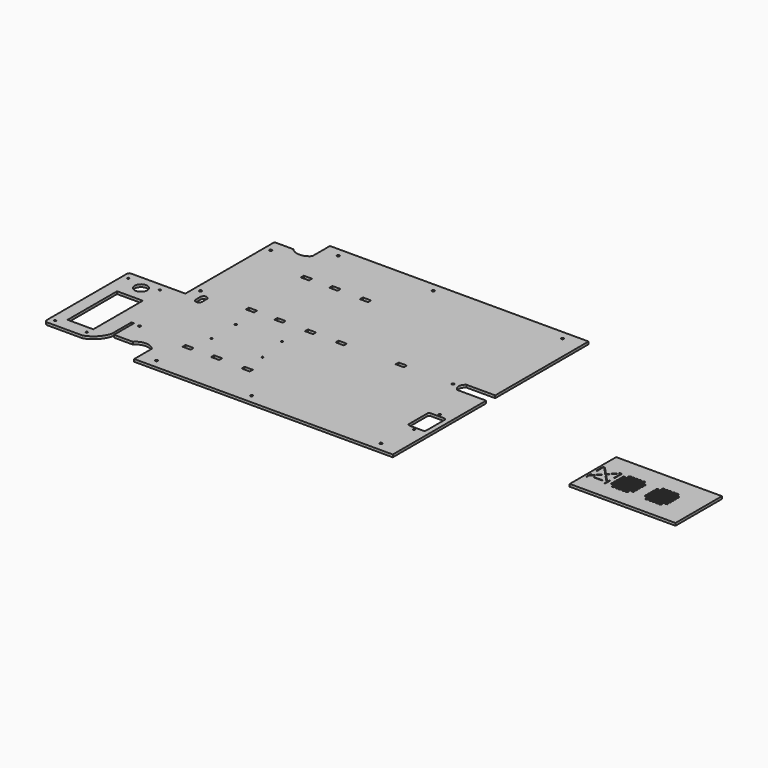
from build123d import *

# Parameters (mm, degrees)
F0_R     = 1.5
F0_R_2   = 2
F0_W     = 40.723241355
F0_H     = 98.1378996708
F0_W_2   = 13
F0_H_2   = 6
F0_R_3   = 10
F1_DEPTH = 4
F0_W_3   = 167.7038488136
F0_H_3   = 92
F0_W_4   = 13.1770956796
F0_H_4   = 1


# Not quite as in the source:
# - a feature names something its author has since deleted; it is built from what else it names


with BuildPart() as f1:
    # F0 (on Top) → F1 (new body)
    with BuildSketch(Plane.XY):
        with BuildLine():
            Line((235, 20), (235, 190))
            Line((235, 190), (235, 194))
            Line((235, 194), (160.2169722319, 194))
            Line((160.2169722319, 194), (-175, 194))
            Line((-175, 194), (-175, 159))
            ThreePointArc((-175, 159), (-190, 152.2242824696), (-205, 159))
            Line((-205, 159), (-235, 159))
            Line((-235, 159), (-235, 18))
            Line((-235, 18), (-235, 0))
            Line((-235, 0), (-235, -17.580891105))
            Line((-235, -17.580891105), (-322.3694663308, -17.580891105))
            ThreePointArc((-322.3694663308, -17.580891105), (-324.1034075985, -19.3986567512), (-324.7344900249, -21.8302322148))
            Line((-324.7344900249, -21.8302322148), (-324.7344900249, -179.7310591129))
            ThreePointArc((-324.7344900249, -179.7310591129), (-323.2700239308, -183.2665930188), (-319.7344900249, -184.7310591129))
            Line((-319.7344900249, -184.7310591129), (-264.2700470778, -184.7310591129))
            ThreePointArc((-264.2700470778, -184.7310591129), (-248.5516048539, -174.8937039891), (-239, -159))
            Line((-239, -159), (-239, -119.5373386145))
            Line((-239, -119.5373386145), (-235, -119.5373386145))
            Line((-235, -119.5373386145), (-235, -141))
            Line((-235, -141), (-235, -141.1135244755))
            Line((-235, -141.1135244755), (-235, -159))
            Line((-235, -159), (-205, -159))
            ThreePointArc((-205, -159), (-190, -152.2242824696), (-175, -159))
            Line((-175, -159), (-175, -194))
            Line((-175, -194), (160.2169722319, -194))
            Line((160.2169722319, -194), (235, -194))
            Line((235, -194), (235, -190))
            Line((235, -190), (235, -20))
            Line((235, -20), (235, -9))
            Line((235, -9), (189.4401907921, -9))
            ThreePointArc((189.4401907921, -9), (184.4617959967, 0), (189.4401907921, 9))
            Line((189.4401907921, 9), (235, 9))
            Line((235, 9), (235, 20))
        make_face()
        with Locations((-315.7939992134, -174.6363174207)):
            Circle(F0_R, mode=Mode.SUBTRACT)
        with Locations((-265.8466312134, -174.8205274207)):
            Circle(F0_R, mode=Mode.SUBTRACT)
        with Locations((-150.6642103195, -180)):
            Circle(F0_R_2, mode=Mode.SUBTRACT)
        with Locations((-284.6316677553, -114.4722954954)):
            Rectangle(F0_W, F0_H, mode=Mode.SUBTRACT)
        with Locations((-225, -121)):
            Circle(F0_R_2, mode=Mode.SUBTRACT)
        with Locations((-142.3513439298, -128.0134530067)):
            Rectangle(F0_W_2, F0_H_2, mode=Mode.SUBTRACT)
        with Locations((-97.480445087, -127.4769221544)):
            Rectangle(F0_W_2, F0_H_2, mode=Mode.SUBTRACT)
        with Locations((0, -180)):
            Circle(F0_R_2, mode=Mode.SUBTRACT)
        with Locations((-48.8024120331, -127.8542791605)):
            Rectangle(F0_W_2, F0_H_2, mode=Mode.SUBTRACT)
        with Locations((-134.561391694, -91.3646608818)):
            Circle(F0_R, mode=Mode.SUBTRACT)
        with Locations((-287.3536279337, -40.1161199984)):
            Circle(F0_R_3, mode=Mode.SUBTRACT)
        with Locations((-315.8466312134, -29.6363174207)):
            Circle(F0_R, mode=Mode.SUBTRACT)
        with Locations((-265.8466312134, -29.6363174207)):
            Circle(F0_R, mode=Mode.SUBTRACT)
        with BuildLine():
            ThreePointArc((-215, -12.7703770995), (-210, -7.7703770995), (-205, -12.7703770995))
            Line((-205, -12.7703770995), (-205, -21.7703770995))
            ThreePointArc((-205, -21.7703770995), (-210, -26.7703770995), (-215, -21.7703770995))
            Line((-215, -21.7703770995), (-215, -12.7703770995))
        make_face(mode=Mode.SUBTRACT)
        with BuildLine():
            ThreePointArc((-223, 0), (-225, -2), (-227, 0))
            ThreePointArc((-227, 0), (-225, 2), (-223, 0))
        make_face(mode=Mode.SUBTRACT)
        with Locations((-134.564578694, -43.3323348818)):
            Circle(F0_R, mode=Mode.SUBTRACT)
        with Locations((-143.6203961174, -0.9194955441)):
            Rectangle(F0_W_2, F0_H_2, mode=Mode.SUBTRACT)
        with Locations((-98.7494972746, -0.3829646918)):
            Rectangle(F0_W_2, F0_H_2, mode=Mode.SUBTRACT)
        with Locations((-53.852118694, -91.0625058818)):
            Circle(F0_R, mode=Mode.SUBTRACT)
        with Locations((-61.225924694, -43.2365928818)):
            Circle(F0_R, mode=Mode.SUBTRACT)
        with Locations((-50.0714642207, -0.7603216978)):
            Rectangle(F0_W_2, F0_H_2, mode=Mode.SUBTRACT)
        with Locations((-1.5765217012, -0.5216977205)):
            Rectangle(F0_W_2, F0_H_2, mode=Mode.SUBTRACT)
        with Locations((205, -180)):
            Circle(F0_R_2, mode=Mode.SUBTRACT)
        with Locations((213.4276428699, -125)):
            Circle(F0_R, mode=Mode.SUBTRACT)
        with BuildLine():
            Line((199.6276428699, -117.6), (199.6276428699, -81.4))
            ThreePointArc((199.6276428699, -81.4), (200.5063225264, -79.2786796564), (202.6276428699, -78.4))
            Line((202.6276428699, -78.4), (224.2276428699, -78.4))
            ThreePointArc((224.2276428699, -78.4), (226.3489632135, -79.2786796564), (227.2276428699, -81.4))
            Line((227.2276428699, -81.4), (227.2276428699, -117.6))
            ThreePointArc((227.2276428699, -117.6), (226.3489632135, -119.7213203436), (224.2276428699, -120.6))
            Line((224.2276428699, -120.6), (202.6276428699, -120.6))
            ThreePointArc((202.6276428699, -120.6), (200.5063225264, -119.7213203436), (199.6276428699, -117.6))
        make_face(mode=Mode.SUBTRACT)
        with Locations((213.4276428699, -74)):
            Circle(F0_R, mode=Mode.SUBTRACT)
        with Locations((175, 0)):
            Circle(F0_R_2, mode=Mode.SUBTRACT)
        with Locations((93.1805941164, 0.1503385957)):
            Rectangle(F0_W_2, F0_H_2, mode=Mode.SUBTRACT)
        with Locations((-225, 139)):
            Circle(F0_R_2, mode=Mode.SUBTRACT)
        with Locations((-143.9774875442, 108.5958170493)):
            Rectangle(F0_W_2, F0_H_2, mode=Mode.SUBTRACT)
        with Locations((-99.1065887014, 109.1323479017)):
            Rectangle(F0_W_2, F0_H_2, mode=Mode.SUBTRACT)
        with Locations((-150.6642103195, 180)):
            Circle(F0_R_2, mode=Mode.SUBTRACT)
        with Locations((-50.4285556475, 108.7549908956)):
            Rectangle(F0_W_2, F0_H_2, mode=Mode.SUBTRACT)
        with Locations((0, 180)):
            Circle(F0_R_2, mode=Mode.SUBTRACT)
        with Locations((205, 180)):
            Circle(F0_R_2, mode=Mode.SUBTRACT)
    extrude(amount=F1_DEPTH)


with BuildPart() as f1b:
    # F0 (on Top) → F1, piece 2 (new body)
    with BuildSketch(Plane.XY):
        with Locations((539.1946978695, -72.6823304409)):
            Rectangle(F0_W_3, F0_H_3)
        with Locations((474.1243227663, -86.1302117599)):
            Rectangle(F0_W_4, F0_H_4, mode=Mode.SUBTRACT)
        Polygon((499.6697502675, -90.1), (500.8244508059, -88.1), (503.1338518827, -88.1), (504.2885524211, -90.1), (503.1338518827, -92.1), (500.8244508059, -92.1), align=None, mode=Mode.SUBTRACT)
        Polygon((470.3372043136, -74.1853925354), (471.1485323172, -74.7817042836), (460.0899253393, -86.6302117599), (460.0899253393, -90.7567794457), (459.0899253393, -90.7567794457), (459.0899253393, -86.2360485793), (459.0899253393, -80.9347892446), (460.0899253393, -80.9347892446), (460.0899253393, -85.1646200079), align=None, mode=Mode.SUBTRACT)
        Polygon((488.0899253393, -86.6302117599), (477.0313183614, -74.7817042836), (477.8426463649, -74.1853925354), (488.0899253393, -85.1646200079), (488.0899253393, -80.9347892446), (489.0899253393, -80.9347892446), (489.0899253393, -86.2360485793), (489.0899253393, -90.7567794457), (488.0899253393, -90.7567794457), align=None, mode=Mode.SUBTRACT)
        Polygon((494.3197502675, -84.75), (495.4744508059, -82.75), (497.7838518827, -82.75), (498.9385524211, -84.75), (497.7838518827, -86.75), (495.4744508059, -86.75), align=None, mode=Mode.SUBTRACT)
        Polygon((499.6697502675, -84.75), (500.8244508059, -82.75), (503.1338518827, -82.75), (504.2885524211, -84.75), (503.1338518827, -86.75), (500.8244508059, -86.75), align=None, mode=Mode.SUBTRACT)
        Polygon((494.3197502675, -79.4), (495.4744508059, -77.4), (497.7838518827, -77.4), (498.9385524211, -79.4), (497.7838518827, -81.4), (495.4744508059, -81.4), align=None, mode=Mode.SUBTRACT)
        Polygon((499.6697502675, -79.4), (500.8244508059, -77.4), (503.1338518827, -77.4), (504.2885524211, -79.4), (503.1338518827, -81.4), (500.8244508059, -81.4), align=None, mode=Mode.SUBTRACT)
        Polygon((494.3197502675, -74.05), (495.4744508059, -72.05), (497.7838518827, -72.05), (498.9385524211, -74.05), (497.7838518827, -76.05), (495.4744508059, -76.05), align=None, mode=Mode.SUBTRACT)
        Polygon((499.6697502675, -74.05), (500.8244508059, -72.05), (503.1338518827, -72.05), (504.2885524211, -74.05), (503.1338518827, -76.05), (500.8244508059, -76.05), align=None, mode=Mode.SUBTRACT)
        with BuildLine():
            Line((474.0899253393, -71.6302117599), (461.8209806075, -58.484913833))
            ThreePointArc((461.8209806075, -58.484913833), (460.7232205999, -58.2368947069), (460.0899253393, -59.1672320834))
            Line((460.0899253393, -59.1672320834), (460.0899253393, -71.6302117599))
            Line((460.0899253393, -71.6302117599), (459.0899253393, -71.6302117599))
            Line((459.0899253393, -71.6302117599), (459.0899253393, -59.1672320834))
            ThreePointArc((459.0899253393, -59.1672320834), (460.3565158605, -57.3065573304), (462.5520358758, -57.8025955827))
            Line((462.5520358758, -57.8025955827), (474.0899253393, -70.1646200079))
            Line((474.0899253393, -70.1646200079), (485.6278148028, -57.8025955827))
            ThreePointArc((485.6278148028, -57.8025955827), (487.823334818, -57.3065573304), (489.0899253393, -59.1672320834))
            Line((489.0899253393, -59.1672320834), (489.0899253393, -71.6302117599))
            Line((489.0899253393, -71.6302117599), (488.0899253393, -71.6302117599))
            Line((488.0899253393, -71.6302117599), (488.0899253393, -59.1672320834))
            ThreePointArc((488.0899253393, -59.1672320834), (487.4566300786, -58.2368947069), (486.358870071, -58.484913833))
            Line((486.358870071, -58.484913833), (474.0899253393, -71.6302117599))
        make_face(mode=Mode.SUBTRACT)
        Polygon((494.3197502675, -68.7), (495.4744508059, -66.7), (497.7838518827, -66.7), (498.9385524211, -68.7), (497.7838518827, -70.7), (495.4744508059, -70.7), align=None, mode=Mode.SUBTRACT)
        Polygon((499.6697502675, -68.7), (500.8244508059, -66.7), (503.1338518827, -66.7), (504.2885524211, -68.7), (503.1338518827, -70.7), (500.8244508059, -70.7), align=None, mode=Mode.SUBTRACT)
        Polygon((494.3197502675, -63.35), (495.4744508059, -61.35), (497.7838518827, -61.35), (498.9385524211, -63.35), (497.7838518827, -65.35), (495.4744508059, -65.35), align=None, mode=Mode.SUBTRACT)
        Polygon((499.6697502675, -63.35), (500.8244508059, -61.35), (503.1338518827, -61.35), (504.2885524211, -63.35), (503.1338518827, -65.35), (500.8244508059, -65.35), align=None, mode=Mode.SUBTRACT)
        Polygon((499.6697502675, -58), (500.8244508059, -56), (503.1338518827, -56), (504.2885524211, -58), (503.1338518827, -60), (500.8244508059, -60), align=None, mode=Mode.SUBTRACT)
        Polygon((505.0197502675, -90.1), (506.1744508059, -88.1), (508.4838518827, -88.1), (509.6385524211, -90.1), (508.4838518827, -92.1), (506.1744508059, -92.1), align=None, mode=Mode.SUBTRACT)
        Polygon((510.3697502675, -90.1), (511.5244508059, -88.1), (513.8338518827, -88.1), (514.9885524211, -90.1), (513.8338518827, -92.1), (511.5244508059, -92.1), align=None, mode=Mode.SUBTRACT)
        Polygon((515.7197502675, -90.1), (516.8744508059, -88.1), (519.1838518827, -88.1), (520.3385524211, -90.1), (519.1838518827, -92.1), (516.8744508059, -92.1), align=None, mode=Mode.SUBTRACT)
        Polygon((521.0697502675, -90.1), (522.2244508059, -88.1), (524.5338518827, -88.1), (525.6885524211, -90.1), (524.5338518827, -92.1), (522.2244508059, -92.1), align=None, mode=Mode.SUBTRACT)
        Polygon((557.1102443947, -91.2547005384), (555.1102443947, -92.4094010768), (553.1102443947, -91.2547005384), (553.1102443947, -88.9452994616), (555.1102443947, -87.7905989232), (557.1102443947, -88.9452994616), align=None, mode=Mode.SUBTRACT)
        Polygon((562.4602443947, -91.2547005384), (560.4602443947, -92.4094010768), (558.4602443947, -91.2547005384), (558.4602443947, -88.9452994616), (560.4602443947, -87.7905989232), (562.4602443947, -88.9452994616), align=None, mode=Mode.SUBTRACT)
        Polygon((505.0197502675, -84.75), (506.1744508059, -82.75), (508.4838518827, -82.75), (509.6385524211, -84.75), (508.4838518827, -86.75), (506.1744508059, -86.75), align=None, mode=Mode.SUBTRACT)
        Polygon((510.3697502675, -84.75), (511.5244508059, -82.75), (513.8338518827, -82.75), (514.9885524211, -84.75), (513.8338518827, -86.75), (511.5244508059, -86.75), align=None, mode=Mode.SUBTRACT)
        Polygon((515.7197502675, -84.75), (516.8744508059, -82.75), (519.1838518827, -82.75), (520.3385524211, -84.75), (519.1838518827, -86.75), (516.8744508059, -86.75), align=None, mode=Mode.SUBTRACT)
        Polygon((505.0197502675, -79.4), (506.1744508059, -77.4), (508.4838518827, -77.4), (509.6385524211, -79.4), (508.4838518827, -81.4), (506.1744508059, -81.4), align=None, mode=Mode.SUBTRACT)
        Polygon((510.3697502675, -79.4), (511.5244508059, -77.4), (513.8338518827, -77.4), (514.9885524211, -79.4), (513.8338518827, -81.4), (511.5244508059, -81.4), align=None, mode=Mode.SUBTRACT)
        Polygon((515.7197502675, -79.4), (516.8744508059, -77.4), (519.1838518827, -77.4), (520.3385524211, -79.4), (519.1838518827, -81.4), (516.8744508059, -81.4), align=None, mode=Mode.SUBTRACT)
        Polygon((521.0697502675, -84.75), (522.2244508059, -82.75), (524.5338518827, -82.75), (525.6885524211, -84.75), (524.5338518827, -86.75), (522.2244508059, -86.75), align=None, mode=Mode.SUBTRACT)
        Polygon((526.4197502675, -84.75), (527.5744508059, -82.75), (529.8838518827, -82.75), (531.0385524211, -84.75), (529.8838518827, -86.75), (527.5744508059, -86.75), align=None, mode=Mode.SUBTRACT)
        Polygon((521.0697502675, -79.4), (522.2244508059, -77.4), (524.5338518827, -77.4), (525.6885524211, -79.4), (524.5338518827, -81.4), (522.2244508059, -81.4), align=None, mode=Mode.SUBTRACT)
        Polygon((526.4197502675, -79.4), (527.5744508059, -77.4), (529.8838518827, -77.4), (531.0385524211, -79.4), (529.8838518827, -81.4), (527.5744508059, -81.4), align=None, mode=Mode.SUBTRACT)
        Polygon((505.0197502675, -74.05), (506.1744508059, -72.05), (508.4838518827, -72.05), (509.6385524211, -74.05), (508.4838518827, -76.05), (506.1744508059, -76.05), align=None, mode=Mode.SUBTRACT)
        Polygon((510.3697502675, -74.05), (511.5244508059, -72.05), (513.8338518827, -72.05), (514.9885524211, -74.05), (513.8338518827, -76.05), (511.5244508059, -76.05), align=None, mode=Mode.SUBTRACT)
        Polygon((515.7197502675, -74.05), (516.8744508059, -72.05), (519.1838518827, -72.05), (520.3385524211, -74.05), (519.1838518827, -76.05), (516.8744508059, -76.05), align=None, mode=Mode.SUBTRACT)
        Polygon((521.0697502675, -74.05), (522.2244508059, -72.05), (524.5338518827, -72.05), (525.6885524211, -74.05), (524.5338518827, -76.05), (522.2244508059, -76.05), align=None, mode=Mode.SUBTRACT)
        Polygon((526.4197502675, -74.05), (527.5744508059, -72.05), (529.8838518827, -72.05), (531.0385524211, -74.05), (529.8838518827, -76.05), (527.5744508059, -76.05), align=None, mode=Mode.SUBTRACT)
        Polygon((551.7602443947, -85.9047005384), (549.7602443947, -87.0594010768), (547.7602443947, -85.9047005384), (547.7602443947, -83.5952994616), (549.7602443947, -82.4405989232), (551.7602443947, -83.5952994616), align=None, mode=Mode.SUBTRACT)
        Polygon((557.1102443947, -85.9047005384), (555.1102443947, -87.0594010768), (553.1102443947, -85.9047005384), (553.1102443947, -83.5952994616), (555.1102443947, -82.4405989232), (557.1102443947, -83.5952994616), align=None, mode=Mode.SUBTRACT)
        Polygon((562.4602443947, -85.9047005384), (560.4602443947, -87.0594010768), (558.4602443947, -85.9047005384), (558.4602443947, -83.5952994616), (560.4602443947, -82.4405989232), (562.4602443947, -83.5952994616), align=None, mode=Mode.SUBTRACT)
        Polygon((551.7602443947, -80.5547005384), (549.7602443947, -81.7094010768), (547.7602443947, -80.5547005384), (547.7602443947, -78.2452994616), (549.7602443947, -77.0905989232), (551.7602443947, -78.2452994616), align=None, mode=Mode.SUBTRACT)
        Polygon((557.1102443947, -80.5547005384), (555.1102443947, -81.7094010768), (553.1102443947, -80.5547005384), (553.1102443947, -78.2452994616), (555.1102443947, -77.0905989232), (557.1102443947, -78.2452994616), align=None, mode=Mode.SUBTRACT)
        Polygon((562.4602443947, -80.5547005384), (560.4602443947, -81.7094010768), (558.4602443947, -80.5547005384), (558.4602443947, -78.2452994616), (560.4602443947, -77.0905989232), (562.4602443947, -78.2452994616), align=None, mode=Mode.SUBTRACT)
        Polygon((551.7602443947, -75.2047005384), (549.7602443947, -76.3594010768), (547.7602443947, -75.2047005384), (547.7602443947, -72.8952994616), (549.7602443947, -71.7405989232), (551.7602443947, -72.8952994616), align=None, mode=Mode.SUBTRACT)
        Polygon((557.1102443947, -75.2047005384), (555.1102443947, -76.3594010768), (553.1102443947, -75.2047005384), (553.1102443947, -72.8952994616), (555.1102443947, -71.7405989232), (557.1102443947, -72.8952994616), align=None, mode=Mode.SUBTRACT)
        Polygon((562.4602443947, -75.2047005384), (560.4602443947, -76.3594010768), (558.4602443947, -75.2047005384), (558.4602443947, -72.8952994616), (560.4602443947, -71.7405989232), (562.4602443947, -72.8952994616), align=None, mode=Mode.SUBTRACT)
        Polygon((567.8102443947, -91.2547005384), (565.8102443947, -92.4094010768), (563.8102443947, -91.2547005384), (563.8102443947, -88.9452994616), (565.8102443947, -87.7905989232), (567.8102443947, -88.9452994616), align=None, mode=Mode.SUBTRACT)
        Polygon((573.1602443947, -91.2547005384), (571.1602443947, -92.4094010768), (569.1602443947, -91.2547005384), (569.1602443947, -88.9452994616), (571.1602443947, -87.7905989232), (573.1602443947, -88.9452994616), align=None, mode=Mode.SUBTRACT)
        Polygon((578.5102443947, -91.2547005384), (576.5102443947, -92.4094010768), (574.5102443947, -91.2547005384), (574.5102443947, -88.9452994616), (576.5102443947, -87.7905989232), (578.5102443947, -88.9452994616), align=None, mode=Mode.SUBTRACT)
        Polygon((567.8102443947, -85.9047005384), (565.8102443947, -87.0594010768), (563.8102443947, -85.9047005384), (563.8102443947, -83.5952994616), (565.8102443947, -82.4405989232), (567.8102443947, -83.5952994616), align=None, mode=Mode.SUBTRACT)
        Polygon((573.1602443947, -85.9047005384), (571.1602443947, -87.0594010768), (569.1602443947, -85.9047005384), (569.1602443947, -83.5952994616), (571.1602443947, -82.4405989232), (573.1602443947, -83.5952994616), align=None, mode=Mode.SUBTRACT)
        Polygon((578.5102443947, -85.9047005384), (576.5102443947, -87.0594010768), (574.5102443947, -85.9047005384), (574.5102443947, -83.5952994616), (576.5102443947, -82.4405989232), (578.5102443947, -83.5952994616), align=None, mode=Mode.SUBTRACT)
        Polygon((567.8102443947, -80.5547005384), (565.8102443947, -81.7094010768), (563.8102443947, -80.5547005384), (563.8102443947, -78.2452994616), (565.8102443947, -77.0905989232), (567.8102443947, -78.2452994616), align=None, mode=Mode.SUBTRACT)
        Polygon((573.1602443947, -80.5547005384), (571.1602443947, -81.7094010768), (569.1602443947, -80.5547005384), (569.1602443947, -78.2452994616), (571.1602443947, -77.0905989232), (573.1602443947, -78.2452994616), align=None, mode=Mode.SUBTRACT)
        Polygon((578.5102443947, -80.5547005384), (576.5102443947, -81.7094010768), (574.5102443947, -80.5547005384), (574.5102443947, -78.2452994616), (576.5102443947, -77.0905989232), (578.5102443947, -78.2452994616), align=None, mode=Mode.SUBTRACT)
        Polygon((583.8602443947, -85.9047005384), (581.8602443947, -87.0594010768), (579.8602443947, -85.9047005384), (579.8602443947, -83.5952994616), (581.8602443947, -82.4405989232), (583.8602443947, -83.5952994616), align=None, mode=Mode.SUBTRACT)
        Polygon((583.8602443947, -80.5547005384), (581.8602443947, -81.7094010768), (579.8602443947, -80.5547005384), (579.8602443947, -78.2452994616), (581.8602443947, -77.0905989232), (583.8602443947, -78.2452994616), align=None, mode=Mode.SUBTRACT)
        Polygon((567.8102443947, -75.2047005384), (565.8102443947, -76.3594010768), (563.8102443947, -75.2047005384), (563.8102443947, -72.8952994616), (565.8102443947, -71.7405989232), (567.8102443947, -72.8952994616), align=None, mode=Mode.SUBTRACT)
        Polygon((573.1602443947, -75.2047005384), (571.1602443947, -76.3594010768), (569.1602443947, -75.2047005384), (569.1602443947, -72.8952994616), (571.1602443947, -71.7405989232), (573.1602443947, -72.8952994616), align=None, mode=Mode.SUBTRACT)
        Polygon((578.5102443947, -75.2047005384), (576.5102443947, -76.3594010768), (574.5102443947, -75.2047005384), (574.5102443947, -72.8952994616), (576.5102443947, -71.7405989232), (578.5102443947, -72.8952994616), align=None, mode=Mode.SUBTRACT)
        Polygon((583.8602443947, -75.2047005384), (581.8602443947, -76.3594010768), (579.8602443947, -75.2047005384), (579.8602443947, -72.8952994616), (581.8602443947, -71.7405989232), (583.8602443947, -72.8952994616), align=None, mode=Mode.SUBTRACT)
        Polygon((505.0197502675, -68.7), (506.1744508059, -66.7), (508.4838518827, -66.7), (509.6385524211, -68.7), (508.4838518827, -70.7), (506.1744508059, -70.7), align=None, mode=Mode.SUBTRACT)
        Polygon((510.3697502675, -68.7), (511.5244508059, -66.7), (513.8338518827, -66.7), (514.9885524211, -68.7), (513.8338518827, -70.7), (511.5244508059, -70.7), align=None, mode=Mode.SUBTRACT)
        Polygon((515.7197502675, -68.7), (516.8744508059, -66.7), (519.1838518827, -66.7), (520.3385524211, -68.7), (519.1838518827, -70.7), (516.8744508059, -70.7), align=None, mode=Mode.SUBTRACT)
        Polygon((521.0697502675, -68.7), (522.2244508059, -66.7), (524.5338518827, -66.7), (525.6885524211, -68.7), (524.5338518827, -70.7), (522.2244508059, -70.7), align=None, mode=Mode.SUBTRACT)
        Polygon((526.4197502675, -68.7), (527.5744508059, -66.7), (529.8838518827, -66.7), (531.0385524211, -68.7), (529.8838518827, -70.7), (527.5744508059, -70.7), align=None, mode=Mode.SUBTRACT)
        Polygon((505.0197502675, -63.35), (506.1744508059, -61.35), (508.4838518827, -61.35), (509.6385524211, -63.35), (508.4838518827, -65.35), (506.1744508059, -65.35), align=None, mode=Mode.SUBTRACT)
        Polygon((510.3697502675, -63.35), (511.5244508059, -61.35), (513.8338518827, -61.35), (514.9885524211, -63.35), (513.8338518827, -65.35), (511.5244508059, -65.35), align=None, mode=Mode.SUBTRACT)
        Polygon((515.7197502675, -63.35), (516.8744508059, -61.35), (519.1838518827, -61.35), (520.3385524211, -63.35), (519.1838518827, -65.35), (516.8744508059, -65.35), align=None, mode=Mode.SUBTRACT)
        Polygon((521.0697502675, -63.35), (522.2244508059, -61.35), (524.5338518827, -61.35), (525.6885524211, -63.35), (524.5338518827, -65.35), (522.2244508059, -65.35), align=None, mode=Mode.SUBTRACT)
        Polygon((526.4197502675, -63.35), (527.5744508059, -61.35), (529.8838518827, -61.35), (531.0385524211, -63.35), (529.8838518827, -65.35), (527.5744508059, -65.35), align=None, mode=Mode.SUBTRACT)
        Polygon((551.7602443947, -69.8547005384), (549.7602443947, -71.0094010768), (547.7602443947, -69.8547005384), (547.7602443947, -67.5452994616), (549.7602443947, -66.3905989232), (551.7602443947, -67.5452994616), align=None, mode=Mode.SUBTRACT)
        Polygon((557.1102443947, -69.8547005384), (555.1102443947, -71.0094010768), (553.1102443947, -69.8547005384), (553.1102443947, -67.5452994616), (555.1102443947, -66.3905989232), (557.1102443947, -67.5452994616), align=None, mode=Mode.SUBTRACT)
        Polygon((562.4602443947, -69.8547005384), (560.4602443947, -71.0094010768), (558.4602443947, -69.8547005384), (558.4602443947, -67.5452994616), (560.4602443947, -66.3905989232), (562.4602443947, -67.5452994616), align=None, mode=Mode.SUBTRACT)
        Polygon((551.7602443947, -64.5047005384), (549.7602443947, -65.6594010768), (547.7602443947, -64.5047005384), (547.7602443947, -62.1952994616), (549.7602443947, -61.0405989232), (551.7602443947, -62.1952994616), align=None, mode=Mode.SUBTRACT)
        Polygon((557.1102443947, -64.5047005384), (555.1102443947, -65.6594010768), (553.1102443947, -64.5047005384), (553.1102443947, -62.1952994616), (555.1102443947, -61.0405989232), (557.1102443947, -62.1952994616), align=None, mode=Mode.SUBTRACT)
        Polygon((562.4602443947, -64.5047005384), (560.4602443947, -65.6594010768), (558.4602443947, -64.5047005384), (558.4602443947, -62.1952994616), (560.4602443947, -61.0405989232), (562.4602443947, -62.1952994616), align=None, mode=Mode.SUBTRACT)
        Polygon((505.0197502675, -58), (506.1744508059, -56), (508.4838518827, -56), (509.6385524211, -58), (508.4838518827, -60), (506.1744508059, -60), align=None, mode=Mode.SUBTRACT)
        Polygon((510.3697502675, -58), (511.5244508059, -56), (513.8338518827, -56), (514.9885524211, -58), (513.8338518827, -60), (511.5244508059, -60), align=None, mode=Mode.SUBTRACT)
        Polygon((515.7197502675, -58), (516.8744508059, -56), (519.1838518827, -56), (520.3385524211, -58), (519.1838518827, -60), (516.8744508059, -60), align=None, mode=Mode.SUBTRACT)
        Polygon((521.0697502675, -58), (522.2244508059, -56), (524.5338518827, -56), (525.6885524211, -58), (524.5338518827, -60), (522.2244508059, -60), align=None, mode=Mode.SUBTRACT)
        Polygon((557.1102443947, -59.1547005384), (555.1102443947, -60.3094010768), (553.1102443947, -59.1547005384), (553.1102443947, -56.8452994616), (555.1102443947, -55.6905989232), (557.1102443947, -56.8452994616), align=None, mode=Mode.SUBTRACT)
        Polygon((562.4602443947, -59.1547005384), (560.4602443947, -60.3094010768), (558.4602443947, -59.1547005384), (558.4602443947, -56.8452994616), (560.4602443947, -55.6905989232), (562.4602443947, -56.8452994616), align=None, mode=Mode.SUBTRACT)
        Polygon((567.8102443947, -69.8547005384), (565.8102443947, -71.0094010768), (563.8102443947, -69.8547005384), (563.8102443947, -67.5452994616), (565.8102443947, -66.3905989232), (567.8102443947, -67.5452994616), align=None, mode=Mode.SUBTRACT)
        Polygon((573.1602443947, -69.8547005384), (571.1602443947, -71.0094010768), (569.1602443947, -69.8547005384), (569.1602443947, -67.5452994616), (571.1602443947, -66.3905989232), (573.1602443947, -67.5452994616), align=None, mode=Mode.SUBTRACT)
        Polygon((578.5102443947, -69.8547005384), (576.5102443947, -71.0094010768), (574.5102443947, -69.8547005384), (574.5102443947, -67.5452994616), (576.5102443947, -66.3905989232), (578.5102443947, -67.5452994616), align=None, mode=Mode.SUBTRACT)
        Polygon((583.8602443947, -69.8547005384), (581.8602443947, -71.0094010768), (579.8602443947, -69.8547005384), (579.8602443947, -67.5452994616), (581.8602443947, -66.3905989232), (583.8602443947, -67.5452994616), align=None, mode=Mode.SUBTRACT)
        Polygon((567.8102443947, -64.5047005384), (565.8102443947, -65.6594010768), (563.8102443947, -64.5047005384), (563.8102443947, -62.1952994616), (565.8102443947, -61.0405989232), (567.8102443947, -62.1952994616), align=None, mode=Mode.SUBTRACT)
        Polygon((573.1602443947, -64.5047005384), (571.1602443947, -65.6594010768), (569.1602443947, -64.5047005384), (569.1602443947, -62.1952994616), (571.1602443947, -61.0405989232), (573.1602443947, -62.1952994616), align=None, mode=Mode.SUBTRACT)
        Polygon((578.5102443947, -64.5047005384), (576.5102443947, -65.6594010768), (574.5102443947, -64.5047005384), (574.5102443947, -62.1952994616), (576.5102443947, -61.0405989232), (578.5102443947, -62.1952994616), align=None, mode=Mode.SUBTRACT)
        Polygon((583.8602443947, -64.5047005384), (581.8602443947, -65.6594010768), (579.8602443947, -64.5047005384), (579.8602443947, -62.1952994616), (581.8602443947, -61.0405989232), (583.8602443947, -62.1952994616), align=None, mode=Mode.SUBTRACT)
        Polygon((567.8102443947, -59.1547005384), (565.8102443947, -60.3094010768), (563.8102443947, -59.1547005384), (563.8102443947, -56.8452994616), (565.8102443947, -55.6905989232), (567.8102443947, -56.8452994616), align=None, mode=Mode.SUBTRACT)
        Polygon((573.1602443947, -59.1547005384), (571.1602443947, -60.3094010768), (569.1602443947, -59.1547005384), (569.1602443947, -56.8452994616), (571.1602443947, -55.6905989232), (573.1602443947, -56.8452994616), align=None, mode=Mode.SUBTRACT)
        Polygon((578.5102443947, -59.1547005384), (576.5102443947, -60.3094010768), (574.5102443947, -59.1547005384), (574.5102443947, -56.8452994616), (576.5102443947, -55.6905989232), (578.5102443947, -56.8452994616), align=None, mode=Mode.SUBTRACT)
    extrude(amount=F1_DEPTH)


solid = Compound([f1.part, f1b.part])
